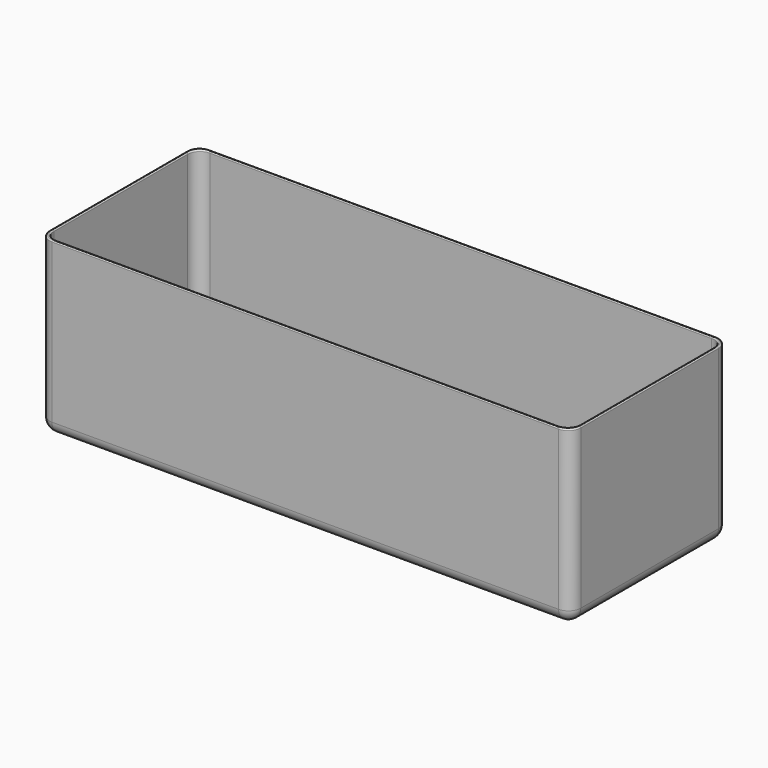
from build123d import *

# Parameters (mm, degrees)
F0_W     = 216
F0_H     = 80
F1_DEPTH = 70
F2_W     = 214
F2_H     = 78
F3_DEPTH = 69
F4_R     = 5
F5_R     = 5
F6_R     = 0.49999


# Not quite as in the source:
# - a fillet or chamfer is up to 0.001 mm smaller than in the source, because OpenCascade refuses the exact size


with BuildPart() as f1:
    # F0 (on Top) → F1 (new body)
    with BuildSketch(Plane.XY):
        Rectangle(F0_W, F0_H)
    extrude(amount=F1_DEPTH)

    # F2 (on face) → F3 (cut)
    with BuildSketch(Plane.XY.offset(70)):
        Rectangle(F2_W, F2_H)
    extrude(amount=-F3_DEPTH, mode=Mode.SUBTRACT)

    # F4
    f4_edges = [f1.edges().sort_by_distance(p)[0] for p in [
        (-107, 39, 35.5),
        (-107, -39, 35.5),
        (107, -39, 35.5),
        (107, 39, 35.5),
        (0, -39, 1),
        (107, 0, 1),
        (0, 39, 1),
        (-107, 0, 1),
        (0, -40, 0),
    ]]
    fillet(f4_edges, radius=F4_R)

    # F5
    f5_edges = [f1.edges().sort_by_distance(p)[0] for p in [
        (0, -40, 5),
        (-108, -40, 37.5),
        (-108, 40, 35),
        (108, 2.5, 0),
        (108, 40, 35),
        (0, 40, 0),
    ]]
    fillet(f5_edges, radius=F5_R)

    # F6 (radius 0.5 in the source; OpenCascade refuses exactly that, so slightly less here)
    f6_edges = [f1.edges().sort_by_distance(p)[0] for p in [
        (0, 40, 70),
        (0, -39, 70),
        (0, 39, 70),
        (107, 0, 70),
        (-105.535534, -37.535534, 70),
        (-107, 0, 70),
        (105.535534, 37.535534, 70),
        (0, -40, 70),
        (108, 0, 70),
        (106.535534, -38.535534, 70),
        (-108, 0, 70),
        (-106.535534, -38.535534, 70),
        (-106.535534, 38.535534, 70),
        (106.535534, 38.535534, 70),
        (105.535534, -37.535534, 70),
        (-105.535534, 37.535534, 70),
    ]]
    fillet(f6_edges, radius=F6_R)


solid = f1.part
